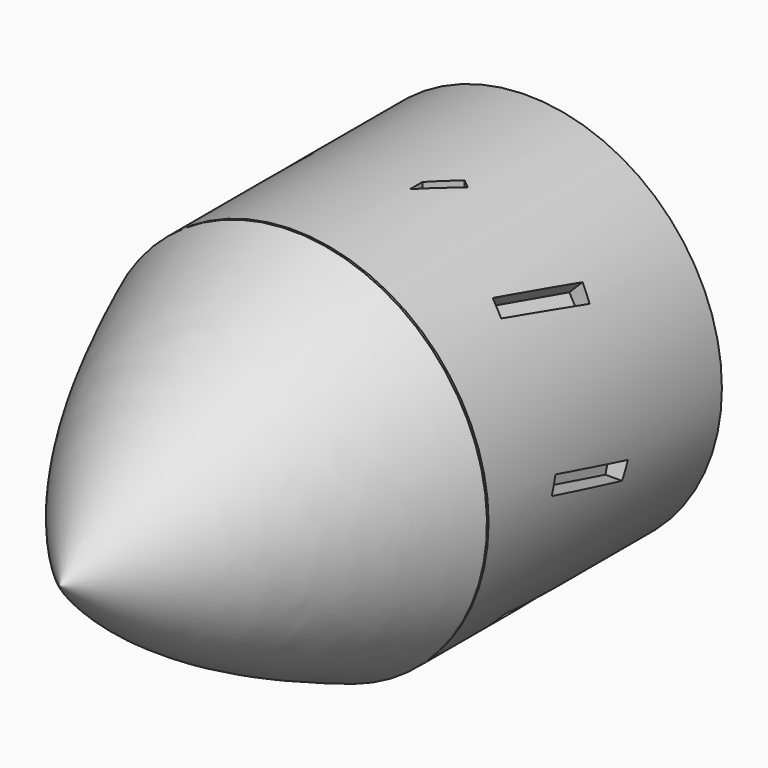
from build123d import *

# Parameters (mm, degrees)
F0_R      = 25.4
F1_DEPTH  = 38.1
F22_DEPTH = 2.54
F23_DEPTH = 2.54
F24_DEPTH = 2.54
F25_DEPTH = 2.54
F26_DEPTH = 2.54
F27_DEPTH = 2.54
F28_DEPTH = 2.54
F29_DEPTH = 2.54


with BuildPart() as f1:
    # F0 (on Front) → F1 (new body)
    with BuildSketch(Plane.XZ):
        Circle(F0_R)
    extrude(amount=F1_DEPTH)

    # F16 (on offset) → F22 (cut)
    with BuildSketch(Plane.YZ.offset(-25.4)):
        Polygon((-27.7622, -1.1684), (-15.83842523, 2.0265658204), (-16.4432335746, 4.2837412912), (-28.3670083446, 1.0887754709), align=None)
    extrude(amount=F22_DEPTH, mode=Mode.SUBTRACT)

    # F15 (on face) → F23 (cut)
    with BuildSketch(Plane(origin=(-17.9605122421, 0, 17.9605122421), x_dir=(0, 1, 0), z_dir=(0.7071067812, 0, -0.7071067812))):
        Polygon((-27.7622, -1.1684), (-15.83842523, 2.0265658204), (-16.4432335746, 4.2837412912), (-28.3670083446, 1.0887754709), align=None)
    extrude(amount=F23_DEPTH, mode=Mode.SUBTRACT)

    # F21 (on offset) → F24 (cut)
    with BuildSketch(Plane.XY.offset(25.4)):
        Polygon((5.9120569609, -17.6502595045), (3.328925729, -21.3393532245), (3.328925729, -23.3763964605), (6.8691542094, -18.3204262127), align=None)
    extrude(amount=-F24_DEPTH, mode=Mode.SUBTRACT)

    # F14 (on face) → F25 (cut)
    with BuildSketch(Plane(origin=(17.9605122421, 0, 17.9605122421), x_dir=(0, 1, 0), z_dir=(0.7071067812, 0, 0.7071067812))):
        Polygon((-27.7622, -1.1684), (-15.83842523, -4.3633658204), (-15.2336168854, -2.1061903495), (-27.1573916554, 1.0887754709), align=None)
    extrude(amount=-F25_DEPTH, mode=Mode.SUBTRACT)

    # F20 (on offset) → F26 (cut)
    with BuildSketch(Plane.YZ.offset(25.4)):
        Polygon((-27.7622, -1.1684), (-15.83842523, -4.3633658204), (-15.2336168854, -2.1061903495), (-27.1573916554, 1.0887754709), align=None)
    extrude(amount=-F26_DEPTH, mode=Mode.SUBTRACT)

    # F19 (on face) → F27 (cut)
    with BuildSketch(Plane(origin=(17.9605122421, 0, -17.9605122421), x_dir=(0, 1, 0), z_dir=(0.7071067812, 0, -0.7071067812))):
        Polygon((-27.7622, -1.1684), (-15.83842523, -4.3633658204), (-15.2336168854, -2.1061903495), (-27.1573916554, 1.0887754709), align=None)
    extrude(amount=-F27_DEPTH, mode=Mode.SUBTRACT)

    # F18 (on offset) → F28 (cut)
    with BuildSketch(Plane.XY.offset(-25.4)):
        Polygon((-4.3633658204, -15.83842523), (-1.1684, -27.7622), (1.0887754709, -27.1573916554), (-2.1061903495, -15.2336168854), align=None)
    extrude(amount=F28_DEPTH, mode=Mode.SUBTRACT)

    # F17 (on face) → F29 (cut)
    with BuildSketch(Plane(origin=(-17.9605122421, 0, -17.9605122421), x_dir=(0, 1, 0), z_dir=(0.7071067812, 0, 0.7071067812))):
        Polygon((-27.7622, -1.1684), (-15.83842523, 2.0265658204), (-16.4432335746, 4.2837412912), (-28.3670083446, 1.0887754709), align=None)
    extrude(amount=F29_DEPTH, mode=Mode.SUBTRACT)


with BuildPart() as f3:
    # F2 (on Right) → F3 (revolve)
    with BuildSketch(Plane.YZ):
        with BuildLine():
            Line((-38.3663102984, 0), (-76.3406405559, 0))
            add(Edge.make_bspline(
                [(-38.3663102984, -25.4), (-54.5826740563, -18.9965814352), (-65.9471228719, -12.1034290642), (-76.3406405559, 0)],
                knots=[0, 0, 0, 0, 45.6859908342, 45.6859908342, 45.6859908342, 45.6859908342], degree=3))
            Line((-38.3663102984, -25.4), (-38.3663102984, 0))
        make_face()
    revolve(axis=Axis((0, -57.3534754272, 0), (0, 1, 0)))


solid = Compound([f1.part, f3.part])
